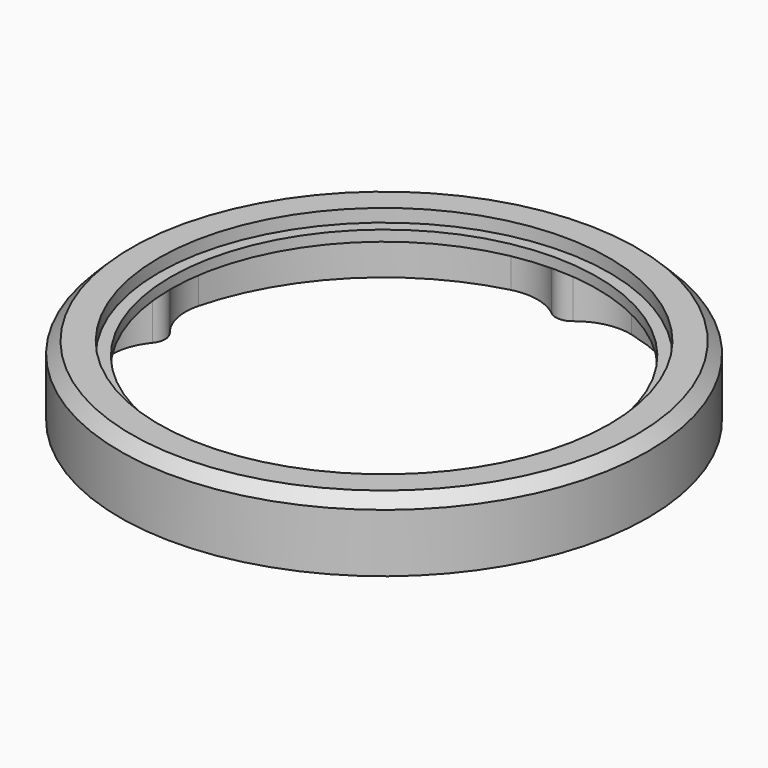
from build123d import *

# Parameters (mm, degrees)
F0_R      = 23.5
F1_DEPTH  = 6.2
F2_T      = -2
F3_SIZE   = 1
F4_R      = 19
F5_DEPTH  = 6.201
F6_R      = 20.05
F7_DEPTH  = 1.15
F8_DEPTH  = 0.1
F9_R      = 1.5
F10_DEPTH = 4.1
F11_R     = 5
F12_R     = 0.8
F13_DEPTH = 4.8


with BuildPart() as f1:
    # F0 (on Top) → F1 (new body)
    with BuildSketch(Plane.XY):
        Circle(F0_R)
    extrude(amount=F1_DEPTH)

    # F2
    f2_openings = [f1.faces().sort_by_distance(p)[0] for p in [
        (0, 0, 0),
    ]]
    offset(amount=F2_T, openings=f2_openings)

    # F3
    f3_edges = [f1.edges().sort_by_distance(p)[0] for p in [
        (-23.5, 0, 6.2),
    ]]
    chamfer(f3_edges, length=F3_SIZE)

    # F4 (on face) → F5 (cut, through all)
    with BuildSketch(Plane.XY.offset(6.2)):
        Circle(F4_R)
    extrude(amount=-F5_DEPTH, mode=Mode.SUBTRACT)

    # F6 (on face) → F7 (cut)
    with BuildSketch(Plane.XY.offset(6.2)):
        Circle(F6_R)
    extrude(amount=-F7_DEPTH, mode=Mode.SUBTRACT)

    # F8 (add): a face of the model
    f8_faces = [f1.faces().sort_by_distance(p)[0] for p in [
        (-20.8918881682, 0, 4.2),
    ]]
    extrude(f8_faces, amount=F8_DEPTH)

    # F9 (on face) → F10 (join, through all)
    with BuildSketch(Plane(origin=(0, 0, 4.1), x_dir=(1, 0, 0), z_dir=(0, 0, -1))):
        with Locations((0, 21)):
            Circle(F9_R)
        with Locations((-21, 0)):
            Circle(F9_R)
        with Locations((0, -21)):
            Circle(F9_R)
        with Locations((21, 0)):
            Circle(F9_R)
    extrude(amount=F10_DEPTH)

    # F11
    f11_edges = [f1.edges().sort_by_distance(p)[0] for p in [
        (21.452381, -1.430158, 2.05),
        (21.452381, 1.430158, 2.05),
        (-1.430158, -21.452381, 2.05),
        (1.430158, -21.452381, 2.05),
        (-21.452381, 1.430158, 2.05),
        (-21.452381, -1.430158, 2.05),
        (-1.430158, 21.452381, 2.05),
        (1.430158, 21.452381, 2.05),
    ]]
    fillet(f11_edges, radius=F11_R)

    # F12 (on face) → F13 (cut)
    with BuildSketch(Plane(origin=(0, 0, 0), x_dir=(1, 0, 0), z_dir=(0, 0, -1))):
        with Locations((0, -21)):
            Circle(F12_R)
        with Locations((21, 0)):
            Circle(F12_R)
        with Locations((0, 21)):
            Circle(F12_R)
        with Locations((-21, 0)):
            Circle(F12_R)
    extrude(amount=-F13_DEPTH, mode=Mode.SUBTRACT)


solid = f1.part
